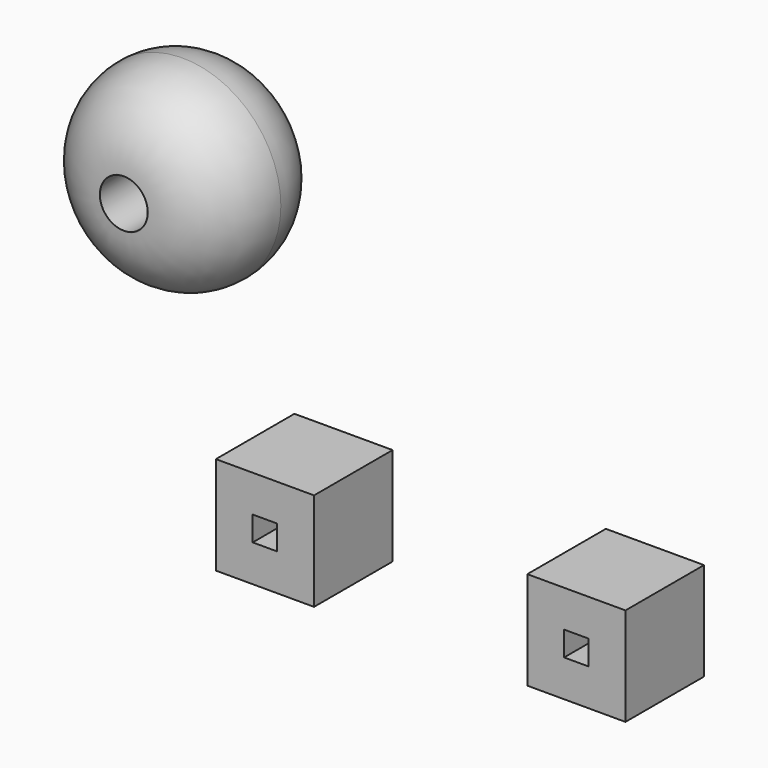
from build123d import *

# Parameters (mm, degrees)
F0_R     = 20
F1_DEPTH = 30
F2_R     = 14.99999
F3_W     = 20
F3_H     = 20
F4_DEPTH = 20
F5_W     = 5
F5_H     = 5
F6_DEPTH = 20
F8_R     = 4.8757387147
F9_DEPTH = 30


# Not quite as in the source:
# - a fillet or chamfer is up to 0.001 mm smaller than in the source, because OpenCascade refuses the exact size


with BuildPart() as f1:
    # F0 (on Front) → F1 (new body)
    with BuildSketch(Plane.XZ):
        with Locations((-52.4842776358, 29.5224059373)):
            Circle(F0_R)
    extrude(amount=F1_DEPTH)

    # F2 (radius 15 in the source; OpenCascade refuses exactly that, so slightly less here)
    f2_edges = [f1.edges().sort_by_distance(p)[0] for p in [
        (-72.484278, -30, 29.522406),
        (-32.484278, -15, 29.522406),
        (-72.484278, 0, 29.522406),
    ]]
    fillet(f2_edges, radius=F2_R)

    # F8 (on face) → F9 (cut)
    with BuildSketch(Plane(origin=(0, 0, 0), x_dir=(-1, 0, 0), z_dir=(0, 1, 0))):
        with Locations((52.4842776358, 29.5224059373)):
            Circle(F8_R)
    extrude(amount=-F9_DEPTH, mode=Mode.SUBTRACT)


with BuildPart() as f4:
    # F3 (on Front) → F4 (new body)
    with BuildSketch(Plane.XZ):
        with Locations((31.7245987244, -26.886938234)):
            Rectangle(F3_W, F3_H)
    extrude(amount=F4_DEPTH)

    # F5 (on face) → F6 (cut)
    with BuildSketch(Plane(origin=(0, 0, 0), x_dir=(-1, 0, 0), z_dir=(0, 1, 0))):
        with Locations((-31.7245987244, -26.886938234)):
            Rectangle(F5_W, F5_H)
    extrude(amount=-F6_DEPTH, mode=Mode.SUBTRACT)


with BuildPart() as f7_1:
    # F7: instance of F4
    add(f4.part.mirror(Plane.YZ))


solid = Compound([f1.part, f4.part, f7_1.part])
